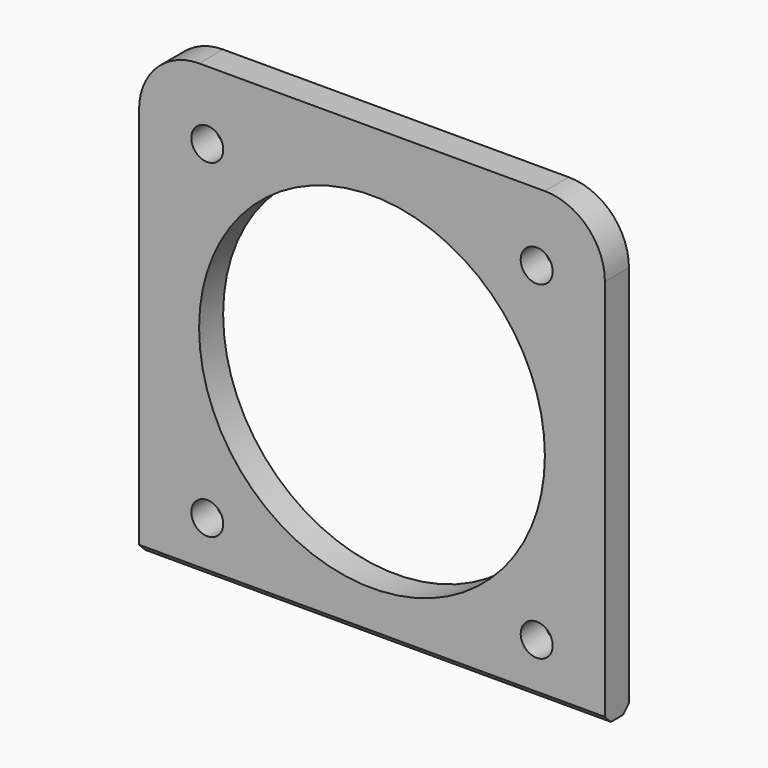
from build123d import *

# Parameters (mm, degrees)
F1_W     = 98.425
F1_H     = 95.25
F1_R     = 36.52774
F2_DEPTH = 6.35
F3_R     = 12.7
F4_SIZE  = 1.5875
F5_D     = 6.7564


# Not quite as in the source:
# - a feature names something its author has since deleted; it is built from what else it names


with BuildPart() as f2:
    # F1 (on face) → F2 (new body)
    with BuildSketch(Plane.XZ):
        with Locations((-208.6903624, 45.950251)):
            Rectangle(F1_W, F1_H)
        Polygon((-169.1837104, 87.1821218), (-168.4475168, 87.1002576), (-167.7522426, 86.8546396), (-167.0979132, 86.4459282), (-166.6073376, 85.9140776), (-165.944296, 85.3010232), (-165.6990082, 84.6054442), (-165.617144, 83.8692252), (-165.617144, 4.8562514), (-165.6990082, 4.1200578), (-165.944296, 3.4251392), (-166.6073376, 2.811399), (-167.0979132, 2.2795484), (-167.7522426, 1.9114516), (-168.4475168, 1.666494), (-169.1837104, 1.5846298), (-248.1557394, 1.5846298), (-248.8919584, 1.666494), (-249.5872072, 1.9114516), (-250.2415366, 2.2795484), (-250.9864424, 2.811399), (-251.395484, 3.4251392), (-251.6407718, 4.1200578), (-251.7226614, 4.8562514), (-251.7226614, 83.8692252), (-251.6407718, 84.6054442), (-251.395484, 85.3010232), (-250.9864424, 85.9140776), (-250.2415366, 86.4459282), (-249.5872072, 86.8546396), (-248.8919584, 87.1002576), (-248.1557394, 87.1821218), align=None, mode=Mode.SUBTRACT)
        Polygon((-167.7522426, 86.8546396), (-168.4475168, 87.1002576), (-169.1837104, 87.1821218), (-248.1557394, 87.1821218), (-248.8919584, 87.1002576), (-249.5872072, 86.8546396), (-250.2415366, 86.4459282), (-250.9864424, 85.9140776), (-251.395484, 85.3010232), (-251.6407718, 84.6054442), (-251.7226614, 83.8692252), (-251.7226614, 4.8562514), (-251.6407718, 4.1200578), (-251.395484, 3.4251392), (-250.9864424, 2.811399), (-250.2415366, 2.2795484), (-249.5872072, 1.9114516), (-248.8919584, 1.666494), (-248.1557394, 1.5846298), (-169.1837104, 1.5846298), (-168.4475168, 1.666494), (-167.7522426, 1.9114516), (-167.0979132, 2.2795484), (-166.6073376, 2.811399), (-165.944296, 3.4251392), (-165.6990082, 4.1200578), (-165.617144, 4.8562514), (-165.617144, 83.8692252), (-165.6990082, 84.6054442), (-165.944296, 85.3010232), (-166.6073376, 85.9140776), (-167.0979132, 86.4459282), align=None)
        with Locations((-208.6903624, 44.362751)):
            Circle(F1_R, mode=Mode.SUBTRACT)
    extrude(amount=F2_DEPTH)

    # F3
    f3_edges = [f2.edges().sort_by_distance(p)[0] for p in [
        (-257.902862, -3.175, 93.575251),
        (-159.477862, -3.175, 93.575251),
    ]]
    fillet(f3_edges, radius=F3_R)

    # F4
    f4_edges = [f2.edges().sort_by_distance(p)[0] for p in [
        (-208.690362, 0, -1.674749),
        (-208.690362, -6.35, -1.674749),
    ]]
    chamfer(f4_edges, length=F4_SIZE)

    # F5 (through all)
    with Locations(Plane(origin=(0, 0, 0), x_dir=(1, 0, 0), z_dir=(0, 1, 0))):
        with Locations((-243.4883624, -79.160751), (-173.8923624, -79.160751), (-173.8923624, -9.564751), (-243.4883624, -9.564751)):
            Hole(F5_D / 2)


solid = f2.part
